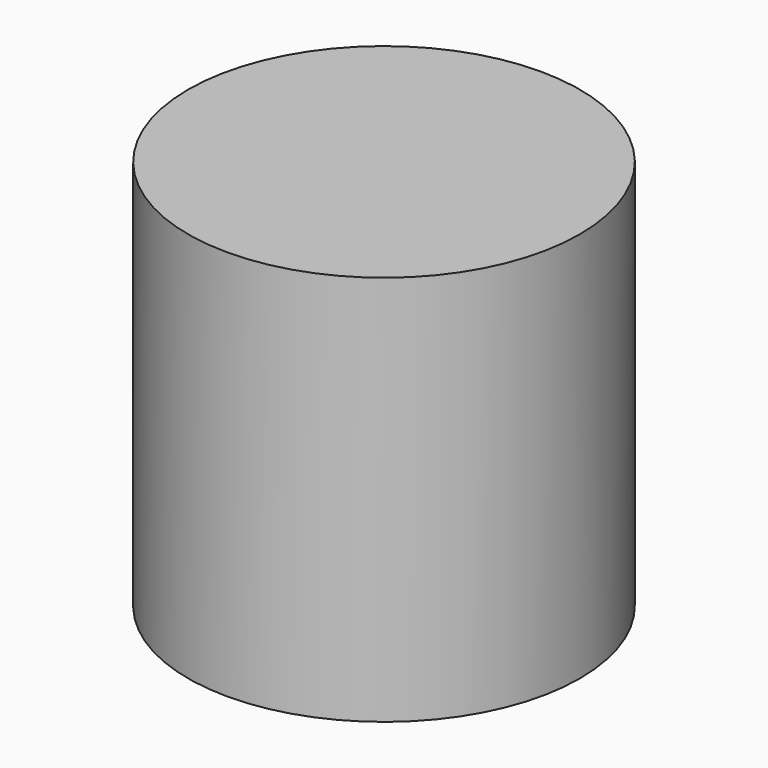
from build123d import *

# Parameters (mm, degrees)
F0_R     = 63.6166007417
F1_DEPTH = 127


# Not quite as in the source:
# - a feature names something its author has since deleted; it is built from what else it names


with BuildPart() as f1:
    # F0 (on Top) → F1 (new body)
    with BuildSketch(Plane.XY):
        with Locations((0, 1.6559939831)):
            Circle(F0_R)
    extrude(amount=-F1_DEPTH)


solid = f1.part
